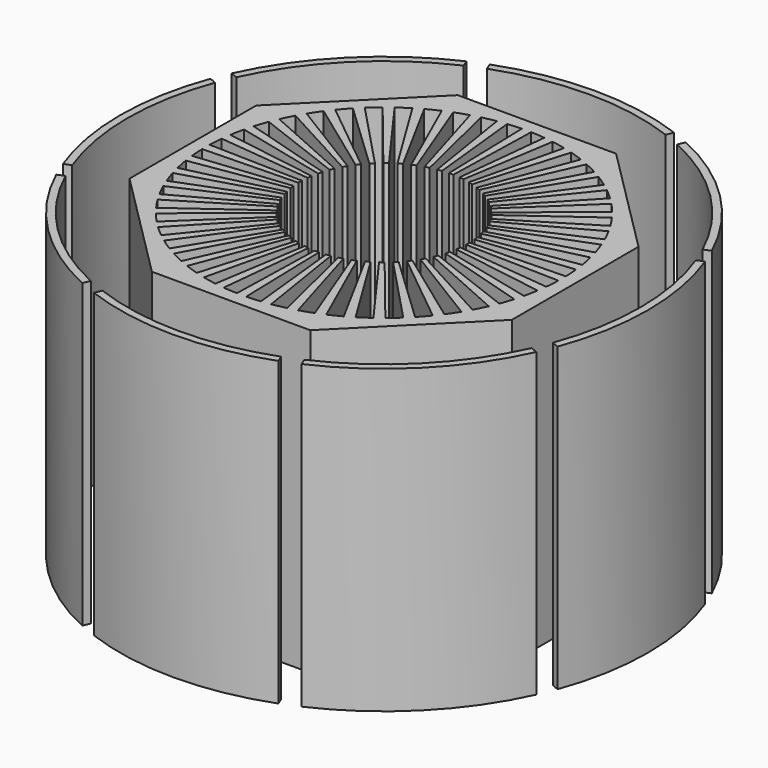
from build123d import *

# Parameters (mm, degrees)
F1_R          = 60
F2_DEPTH      = 50.8
F4_DEPTH      = 50.8
F4_DEPTH_BACK = 50.8
F7_DEPTH      = 50.8
F7_DEPTH_BACK = 50.8
F8_COUNT      = 8


with BuildPart() as f2:
    # F1 (on Top) → F2 (new body, symmetric)
    with BuildSketch(Plane.XY):
        Polygon((26.67, 64.3870757085), (-26.67, 64.3870757085), (-64.3870757085, 26.67), (-64.3870757085, -26.67), (-26.67, -64.3870757085), (26.67, -64.3870757085), (64.3870757085, -26.67), (64.3870757085, 26.67), align=None)
        Circle(F1_R, mode=Mode.SUBTRACT)
    extrude(amount=F2_DEPTH, both=True)

    # F3 (on Top) → F4 (join, two sides)
    with BuildSketch(Plane.XY) as f4_sk:
        with BuildLine():
            ThreePointArc((-0.7394987897, 28.2403194306), (0, 28.25), (0.7394987897, 28.2403194306))
            Line((0.7394987897, 28.2403194306), (1.5706168985, 59.9794394985))
            ThreePointArc((1.5706168985, 59.9794394985), (0, 60), (-1.5706168985, 59.9794394985))
            Line((-1.5706168985, 59.9794394985), (-0.7394987897, 28.2403194306))
        make_face()
        with BuildLine():
            Line((-9.3860679024, 59.2613004357), (-4.4192736374, 27.9021956218))
            ThreePointArc((-4.4192736374, 27.9021956218), (-3.6873649302, 28.0083173338), (-2.9529290873, 28.0952435442))
            Line((-2.9529290873, 28.0952435442), (-6.2717077961, 59.6713137221))
            ThreePointArc((-6.2717077961, 59.6713137221), (-7.8315715332, 59.4866916824), (-9.3860679024, 59.2613004357))
        make_face()
        with BuildLine():
            Line((-17.0409206822, 57.5291840921), (-8.0234334879, 27.08665751))
            ThreePointArc((-8.0234334879, 27.08665751), (-7.3116380241, 27.2874045927), (-6.5948315289, 27.4694502512))
            Line((-6.5948315289, 27.4694502512), (-14.0067218314, 58.3421952239))
            ThreePointArc((-14.0067218314, 58.3421952239), (-15.5291427062, 57.9555495773), (-17.0409206822, 57.5291840921))
        make_face()
        with BuildLine():
            Line((-24.4041985845, 54.8127274586), (-11.4903101669, 25.8076591784))
            ThreePointArc((-11.4903101669, 25.8076591784), (-10.8108069643, 26.0995967934), (-10.1238945747, 26.3736470485))
            Line((-10.1238945747, 26.3736470485), (-21.5020769727, 56.0148255898))
            ThreePointArc((-21.5020769727, 56.0148255898), (-22.9610059419, 55.4327719507), (-24.4041985845, 54.8127274586))
        make_face()
        with BuildLine():
            Line((-31.349913883, 51.1584098612), (-14.7605844532, 24.087084643))
            ThreePointArc((-14.7605844532, 24.087084643), (-14.125, 24.4652176569), (-13.4797349773, 24.8265834327))
            Line((-13.4797349773, 24.8265834327), (-28.6295256156, 52.7290267597))
            ThreePointArc((-28.6295256156, 52.7290267597), (-30, 51.9615242271), (-31.349913883, 51.1584098612))
        make_face()
        with BuildLine():
            Line((-37.759223463, 46.6287576874), (-17.7783010472, 21.9543734112))
            ThreePointArc((-17.7783010472, 21.9543734112), (-17.1975103695, 22.4122318632), (-16.6049333773, 22.8547300911))
            Line((-16.6049333773, 22.8547300911), (-35.2671151375, 48.5410196625))
            ThreePointArc((-35.2671151375, 48.5410196625), (-36.5256857405, 47.6012004175), (-37.759223463, 46.6287576874))
        make_face()
        with BuildLine():
            Line((-43.5224622607, 41.3012745416), (-20.4918259811, 19.4460167633))
            ThreePointArc((-20.4918259811, 19.4460167633), (-19.9757665685, 19.9757665685), (-19.4460167633, 20.4918259811))
            Line((-19.4460167633, 20.4918259811), (-41.3012745416, 43.5224622607))
            ThreePointArc((-41.3012745416, 43.5224622607), (-42.4264068712, 42.4264068712), (-43.5224622607, 41.3012745416))
        make_face()
        with BuildLine():
            Line((-48.5410196625, 35.2671151375), (-22.8547300911, 16.6049333773))
            ThreePointArc((-22.8547300911, 16.6049333773), (-22.4122318632, 17.1975103695), (-21.9543734112, 17.7783010472))
            Line((-21.9543734112, 17.7783010472), (-46.6287576874, 37.759223463))
            ThreePointArc((-46.6287576874, 37.759223463), (-47.6012004175, 36.5256857405), (-48.5410196625, 35.2671151375))
        make_face()
        with BuildLine():
            Line((-52.7290267597, 28.6295256156), (-24.8265834327, 13.4797349773))
            ThreePointArc((-24.8265834327, 13.4797349773), (-24.4652176569, 14.125), (-24.087084643, 14.7605844532))
            Line((-24.087084643, 14.7605844532), (-51.1584098612, 31.349913883))
            ThreePointArc((-51.1584098612, 31.349913883), (-51.9615242271, 30), (-52.7290267597, 28.6295256156))
        make_face()
        with BuildLine():
            Line((-56.0148255898, 21.5020769727), (-26.3736470485, 10.1238945747))
            ThreePointArc((-26.3736470485, 10.1238945747), (-26.0995967934, 10.8108069643), (-25.8076591784, 11.4903101669))
            Line((-25.8076591784, 11.4903101669), (-54.8127274586, 24.4041985845))
            ThreePointArc((-54.8127274586, 24.4041985845), (-55.4327719507, 22.9610059419), (-56.0148255898, 21.5020769727))
        make_face()
        with BuildLine():
            Line((-58.3421952239, 14.0067218314), (-27.4694502512, 6.5948315289))
            ThreePointArc((-27.4694502512, 6.5948315289), (-27.2874045927, 7.3116380241), (-27.08665751, 8.0234334879))
            Line((-27.08665751, 8.0234334879), (-57.5291840921, 17.0409206822))
            ThreePointArc((-57.5291840921, 17.0409206822), (-57.9555495773, 15.5291427062), (-58.3421952239, 14.0067218314))
        make_face()
        with BuildLine():
            Line((-59.6713137221, 6.2717077961), (-28.0952435442, 2.9529290873))
            ThreePointArc((-28.0952435442, 2.9529290873), (-28.0083173338, 3.6873649302), (-27.9021956218, 4.4192736374))
            Line((-27.9021956218, 4.4192736374), (-59.2613004357, 9.3860679024))
            ThreePointArc((-59.2613004357, 9.3860679024), (-59.4866916824, 7.8315715332), (-59.6713137221, 6.2717077961))
        make_face()
        with BuildLine():
            Line((-59.9794394985, -1.5706168985), (-28.2403194306, -0.7394987897))
            ThreePointArc((-28.2403194306, -0.7394987897), (-28.25, 0), (-28.2403194306, 0.7394987897))
            Line((-28.2403194306, 0.7394987897), (-59.9794394985, 1.5706168985))
            ThreePointArc((-59.9794394985, 1.5706168985), (-60, 0), (-59.9794394985, -1.5706168985))
        make_face()
        with BuildLine():
            Line((-59.2613004357, -9.3860679024), (-27.9021956218, -4.4192736374))
            ThreePointArc((-27.9021956218, -4.4192736374), (-28.0083173338, -3.6873649302), (-28.0952435442, -2.9529290873))
            Line((-28.0952435442, -2.9529290873), (-59.6713137221, -6.2717077961))
            ThreePointArc((-59.6713137221, -6.2717077961), (-59.4866916824, -7.8315715332), (-59.2613004357, -9.3860679024))
        make_face()
        with BuildLine():
            Line((-57.5291840921, -17.0409206822), (-27.08665751, -8.0234334879))
            ThreePointArc((-27.08665751, -8.0234334879), (-27.2874045927, -7.3116380241), (-27.4694502512, -6.5948315289))
            Line((-27.4694502512, -6.5948315289), (-58.3421952239, -14.0067218314))
            ThreePointArc((-58.3421952239, -14.0067218314), (-57.9555495773, -15.5291427062), (-57.5291840921, -17.0409206822))
        make_face()
        with BuildLine():
            Line((-54.8127274586, -24.4041985845), (-25.8076591784, -11.4903101669))
            ThreePointArc((-25.8076591784, -11.4903101669), (-26.0995967934, -10.8108069643), (-26.3736470485, -10.1238945747))
            Line((-26.3736470485, -10.1238945747), (-56.0148255898, -21.5020769727))
            ThreePointArc((-56.0148255898, -21.5020769727), (-55.4327719507, -22.9610059419), (-54.8127274586, -24.4041985845))
        make_face()
        with BuildLine():
            Line((-51.1584098612, -31.349913883), (-24.087084643, -14.7605844532))
            ThreePointArc((-24.087084643, -14.7605844532), (-24.4652176569, -14.125), (-24.8265834327, -13.4797349773))
            Line((-24.8265834327, -13.4797349773), (-52.7290267597, -28.6295256156))
            ThreePointArc((-52.7290267597, -28.6295256156), (-51.9615242271, -30), (-51.1584098612, -31.349913883))
        make_face()
        with BuildLine():
            Line((-46.6287576874, -37.759223463), (-21.9543734112, -17.7783010472))
            ThreePointArc((-21.9543734112, -17.7783010472), (-22.4122318632, -17.1975103695), (-22.8547300911, -16.6049333773))
            Line((-22.8547300911, -16.6049333773), (-48.5410196625, -35.2671151375))
            ThreePointArc((-48.5410196625, -35.2671151375), (-47.6012004175, -36.5256857405), (-46.6287576874, -37.759223463))
        make_face()
        with BuildLine():
            Line((-41.3012745416, -43.5224622607), (-19.4460167633, -20.4918259811))
            ThreePointArc((-19.4460167633, -20.4918259811), (-19.9757665685, -19.9757665685), (-20.4918259811, -19.4460167633))
            Line((-20.4918259811, -19.4460167633), (-43.5224622607, -41.3012745416))
            ThreePointArc((-43.5224622607, -41.3012745416), (-42.4264068712, -42.4264068712), (-41.3012745416, -43.5224622607))
        make_face()
        with BuildLine():
            Line((-35.2671151375, -48.5410196625), (-16.6049333773, -22.8547300911))
            ThreePointArc((-16.6049333773, -22.8547300911), (-17.1975103695, -22.4122318632), (-17.7783010472, -21.9543734112))
            Line((-17.7783010472, -21.9543734112), (-37.759223463, -46.6287576874))
            ThreePointArc((-37.759223463, -46.6287576874), (-36.5256857405, -47.6012004175), (-35.2671151375, -48.5410196625))
        make_face()
        with BuildLine():
            Line((-28.6295256156, -52.7290267597), (-13.4797349773, -24.8265834327))
            ThreePointArc((-13.4797349773, -24.8265834327), (-14.125, -24.4652176569), (-14.7605844532, -24.087084643))
            Line((-14.7605844532, -24.087084643), (-31.349913883, -51.1584098612))
            ThreePointArc((-31.349913883, -51.1584098612), (-30, -51.9615242271), (-28.6295256156, -52.7290267597))
        make_face()
        with BuildLine():
            Line((-21.5020769727, -56.0148255898), (-10.1238945747, -26.3736470485))
            ThreePointArc((-10.1238945747, -26.3736470485), (-10.8108069643, -26.0995967934), (-11.4903101669, -25.8076591784))
            Line((-11.4903101669, -25.8076591784), (-24.4041985845, -54.8127274586))
            ThreePointArc((-24.4041985845, -54.8127274586), (-22.9610059419, -55.4327719507), (-21.5020769727, -56.0148255898))
        make_face()
        with BuildLine():
            Line((-14.0067218314, -58.3421952239), (-6.5948315289, -27.4694502512))
            ThreePointArc((-6.5948315289, -27.4694502512), (-7.3116380241, -27.2874045927), (-8.0234334879, -27.08665751))
            Line((-8.0234334879, -27.08665751), (-17.0409206822, -57.5291840921))
            ThreePointArc((-17.0409206822, -57.5291840921), (-15.5291427062, -57.9555495773), (-14.0067218314, -58.3421952239))
        make_face()
        with BuildLine():
            Line((-6.2717077961, -59.6713137221), (-2.9529290873, -28.0952435442))
            ThreePointArc((-2.9529290873, -28.0952435442), (-3.6873649302, -28.0083173338), (-4.4192736374, -27.9021956218))
            Line((-4.4192736374, -27.9021956218), (-9.3860679024, -59.2613004357))
            ThreePointArc((-9.3860679024, -59.2613004357), (-7.8315715332, -59.4866916824), (-6.2717077961, -59.6713137221))
        make_face()
        with BuildLine():
            Line((1.5706168985, -59.9794394985), (0.7394987897, -28.2403194306))
            ThreePointArc((0.7394987897, -28.2403194306), (0, -28.25), (-0.7394987897, -28.2403194306))
            Line((-0.7394987897, -28.2403194306), (-1.5706168985, -59.9794394985))
            ThreePointArc((-1.5706168985, -59.9794394985), (0, -60), (1.5706168985, -59.9794394985))
        make_face()
        with BuildLine():
            Line((9.3860679024, -59.2613004357), (4.4192736374, -27.9021956218))
            ThreePointArc((4.4192736374, -27.9021956218), (3.6873649302, -28.0083173338), (2.9529290873, -28.0952435442))
            Line((2.9529290873, -28.0952435442), (6.2717077961, -59.6713137221))
            ThreePointArc((6.2717077961, -59.6713137221), (7.8315715332, -59.4866916824), (9.3860679024, -59.2613004357))
        make_face()
        with BuildLine():
            Line((17.0409206822, -57.5291840921), (8.0234334879, -27.08665751))
            ThreePointArc((8.0234334879, -27.08665751), (7.3116380241, -27.2874045927), (6.5948315289, -27.4694502512))
            Line((6.5948315289, -27.4694502512), (14.0067218314, -58.3421952239))
            ThreePointArc((14.0067218314, -58.3421952239), (15.5291427062, -57.9555495773), (17.0409206822, -57.5291840921))
        make_face()
        with BuildLine():
            Line((24.4041985845, -54.8127274586), (11.4903101669, -25.8076591784))
            ThreePointArc((11.4903101669, -25.8076591784), (10.8108069643, -26.0995967934), (10.1238945747, -26.3736470485))
            Line((10.1238945747, -26.3736470485), (21.5020769727, -56.0148255898))
            ThreePointArc((21.5020769727, -56.0148255898), (22.9610059419, -55.4327719507), (24.4041985845, -54.8127274586))
        make_face()
        with BuildLine():
            Line((31.349913883, -51.1584098612), (14.7605844532, -24.087084643))
            ThreePointArc((14.7605844532, -24.087084643), (14.125, -24.4652176569), (13.4797349773, -24.8265834327))
            Line((13.4797349773, -24.8265834327), (28.6295256156, -52.7290267597))
            ThreePointArc((28.6295256156, -52.7290267597), (30, -51.9615242271), (31.349913883, -51.1584098612))
        make_face()
        with BuildLine():
            Line((37.759223463, -46.6287576874), (17.7783010472, -21.9543734112))
            ThreePointArc((17.7783010472, -21.9543734112), (17.1975103695, -22.4122318632), (16.6049333773, -22.8547300911))
            Line((16.6049333773, -22.8547300911), (35.2671151375, -48.5410196625))
            ThreePointArc((35.2671151375, -48.5410196625), (36.5256857405, -47.6012004175), (37.759223463, -46.6287576874))
        make_face()
        with BuildLine():
            Line((43.5224622607, -41.3012745416), (20.4918259811, -19.4460167633))
            ThreePointArc((20.4918259811, -19.4460167633), (19.9757665685, -19.9757665685), (19.4460167633, -20.4918259811))
            Line((19.4460167633, -20.4918259811), (41.3012745416, -43.5224622607))
            ThreePointArc((41.3012745416, -43.5224622607), (42.4264068712, -42.4264068712), (43.5224622607, -41.3012745416))
        make_face()
        with BuildLine():
            Line((48.5410196625, -35.2671151375), (22.8547300911, -16.6049333773))
            ThreePointArc((22.8547300911, -16.6049333773), (22.4122318632, -17.1975103695), (21.9543734112, -17.7783010472))
            Line((21.9543734112, -17.7783010472), (46.6287576874, -37.759223463))
            ThreePointArc((46.6287576874, -37.759223463), (47.6012004175, -36.5256857405), (48.5410196625, -35.2671151375))
        make_face()
        with BuildLine():
            Line((52.7290267597, -28.6295256156), (24.8265834327, -13.4797349773))
            ThreePointArc((24.8265834327, -13.4797349773), (24.4652176569, -14.125), (24.087084643, -14.7605844532))
            Line((24.087084643, -14.7605844532), (51.1584098612, -31.349913883))
            ThreePointArc((51.1584098612, -31.349913883), (51.9615242271, -30), (52.7290267597, -28.6295256156))
        make_face()
        with BuildLine():
            Line((56.0148255898, -21.5020769727), (26.3736470485, -10.1238945747))
            ThreePointArc((26.3736470485, -10.1238945747), (26.0995967934, -10.8108069643), (25.8076591784, -11.4903101669))
            Line((25.8076591784, -11.4903101669), (54.8127274586, -24.4041985845))
            ThreePointArc((54.8127274586, -24.4041985845), (55.4327719507, -22.9610059419), (56.0148255898, -21.5020769727))
        make_face()
        with BuildLine():
            Line((58.3421952239, -14.0067218314), (27.4694502512, -6.5948315289))
            ThreePointArc((27.4694502512, -6.5948315289), (27.2874045927, -7.3116380241), (27.08665751, -8.0234334879))
            Line((27.08665751, -8.0234334879), (57.5291840921, -17.0409206822))
            ThreePointArc((57.5291840921, -17.0409206822), (57.9555495773, -15.5291427062), (58.3421952239, -14.0067218314))
        make_face()
        with BuildLine():
            Line((59.6713137221, -6.2717077961), (28.0952435442, -2.9529290873))
            ThreePointArc((28.0952435442, -2.9529290873), (28.0083173338, -3.6873649302), (27.9021956218, -4.4192736374))
            Line((27.9021956218, -4.4192736374), (59.2613004357, -9.3860679024))
            ThreePointArc((59.2613004357, -9.3860679024), (59.4866916824, -7.8315715332), (59.6713137221, -6.2717077961))
        make_face()
        with BuildLine():
            Line((59.9794394985, 1.5706168985), (28.2403194306, 0.7394987897))
            ThreePointArc((28.2403194306, 0.7394987897), (28.25, 0), (28.2403194306, -0.7394987897))
            Line((28.2403194306, -0.7394987897), (59.9794394985, -1.5706168985))
            ThreePointArc((59.9794394985, -1.5706168985), (60, 0), (59.9794394985, 1.5706168985))
        make_face()
        with BuildLine():
            Line((59.2613004357, 9.3860679024), (27.9021956218, 4.4192736374))
            ThreePointArc((27.9021956218, 4.4192736374), (28.0083173338, 3.6873649302), (28.0952435442, 2.9529290873))
            Line((28.0952435442, 2.9529290873), (59.6713137221, 6.2717077961))
            ThreePointArc((59.6713137221, 6.2717077961), (59.4866916824, 7.8315715332), (59.2613004357, 9.3860679024))
        make_face()
        with BuildLine():
            Line((57.5291840921, 17.0409206822), (27.08665751, 8.0234334879))
            ThreePointArc((27.08665751, 8.0234334879), (27.2874045927, 7.3116380241), (27.4694502512, 6.5948315289))
            Line((27.4694502512, 6.5948315289), (58.3421952239, 14.0067218314))
            ThreePointArc((58.3421952239, 14.0067218314), (57.9555495773, 15.5291427062), (57.5291840921, 17.0409206822))
        make_face()
        with BuildLine():
            Line((54.8127274586, 24.4041985845), (25.8076591784, 11.4903101669))
            ThreePointArc((25.8076591784, 11.4903101669), (26.0995967934, 10.8108069643), (26.3736470485, 10.1238945747))
            Line((26.3736470485, 10.1238945747), (56.0148255898, 21.5020769727))
            ThreePointArc((56.0148255898, 21.5020769727), (55.4327719507, 22.9610059419), (54.8127274586, 24.4041985845))
        make_face()
        with BuildLine():
            Line((51.1584098612, 31.349913883), (24.087084643, 14.7605844532))
            ThreePointArc((24.087084643, 14.7605844532), (24.4652176569, 14.125), (24.8265834327, 13.4797349773))
            Line((24.8265834327, 13.4797349773), (52.7290267597, 28.6295256156))
            ThreePointArc((52.7290267597, 28.6295256156), (51.9615242271, 30), (51.1584098612, 31.349913883))
        make_face()
        with BuildLine():
            Line((46.6287576874, 37.759223463), (21.9543734112, 17.7783010472))
            ThreePointArc((21.9543734112, 17.7783010472), (22.4122318632, 17.1975103695), (22.8547300911, 16.6049333773))
            Line((22.8547300911, 16.6049333773), (48.5410196625, 35.2671151375))
            ThreePointArc((48.5410196625, 35.2671151375), (47.6012004175, 36.5256857405), (46.6287576874, 37.759223463))
        make_face()
        with BuildLine():
            Line((41.3012745416, 43.5224622607), (19.4460167633, 20.4918259811))
            ThreePointArc((19.4460167633, 20.4918259811), (19.9757665685, 19.9757665685), (20.4918259811, 19.4460167633))
            Line((20.4918259811, 19.4460167633), (43.5224622607, 41.3012745416))
            ThreePointArc((43.5224622607, 41.3012745416), (42.4264068712, 42.4264068712), (41.3012745416, 43.5224622607))
        make_face()
        with BuildLine():
            Line((35.2671151375, 48.5410196625), (16.6049333773, 22.8547300911))
            ThreePointArc((16.6049333773, 22.8547300911), (17.1975103695, 22.4122318632), (17.7783010472, 21.9543734112))
            Line((17.7783010472, 21.9543734112), (37.759223463, 46.6287576874))
            ThreePointArc((37.759223463, 46.6287576874), (36.5256857405, 47.6012004175), (35.2671151375, 48.5410196625))
        make_face()
        with BuildLine():
            Line((28.6295256156, 52.7290267597), (13.4797349773, 24.8265834327))
            ThreePointArc((13.4797349773, 24.8265834327), (14.125, 24.4652176569), (14.7605844532, 24.087084643))
            Line((14.7605844532, 24.087084643), (31.349913883, 51.1584098612))
            ThreePointArc((31.349913883, 51.1584098612), (30, 51.9615242271), (28.6295256156, 52.7290267597))
        make_face()
        with BuildLine():
            Line((21.5020769727, 56.0148255898), (10.1238945747, 26.3736470485))
            ThreePointArc((10.1238945747, 26.3736470485), (10.8108069643, 26.0995967934), (11.4903101669, 25.8076591784))
            Line((11.4903101669, 25.8076591784), (24.4041985845, 54.8127274586))
            ThreePointArc((24.4041985845, 54.8127274586), (22.9610059419, 55.4327719507), (21.5020769727, 56.0148255898))
        make_face()
        with BuildLine():
            Line((14.0067218314, 58.3421952239), (6.5948315289, 27.4694502512))
            ThreePointArc((6.5948315289, 27.4694502512), (7.3116380241, 27.2874045927), (8.0234334879, 27.08665751))
            Line((8.0234334879, 27.08665751), (17.0409206822, 57.5291840921))
            ThreePointArc((17.0409206822, 57.5291840921), (15.5291427062, 57.9555495773), (14.0067218314, 58.3421952239))
        make_face()
        with BuildLine():
            Line((6.2717077961, 59.6713137221), (2.9529290873, 28.0952435442))
            ThreePointArc((2.9529290873, 28.0952435442), (3.6873649302, 28.0083173338), (4.4192736374, 27.9021956218))
            Line((4.4192736374, 27.9021956218), (9.3860679024, 59.2613004357))
            ThreePointArc((9.3860679024, 59.2613004357), (7.8315715332, 59.4866916824), (6.2717077961, 59.6713137221))
        make_face()
    extrude(amount=F4_DEPTH)
    extrude(f4_sk.sketch, amount=-F4_DEPTH_BACK)


with BuildPart() as f7:
    # F6 (on Top) → F7 (new body, two sides)
    with BuildSketch(Plane.XY) as f7_sk:
        with BuildLine():
            Line((-30.0928812264, -80.9473168147), (-31.0655359146, -83.2955129544))
            ThreePointArc((-31.0655359146, -83.2955129544), (0, -88.9), (31.0655359146, -83.2955129544))
            Line((31.0655359146, -83.2955129544), (30.0928812264, -80.9473168147))
            ThreePointArc((30.0928812264, -80.9473168147), (0, -86.36), (-30.0928812264, -80.9473168147))
        make_face()
    extrude(amount=-F7_DEPTH)
    extrude(f7_sk.sketch, amount=F7_DEPTH_BACK)


with BuildPart() as f8_1:
    # F8: instance of F7
    add(f7.part.rotate(Axis((0, 0, 0), (0, 0, 1)), 1 * 360 / F8_COUNT))


with BuildPart() as f8_2:
    # F8: instance of F7
    add(f7.part.rotate(Axis((0, 0, 0), (0, 0, 1)), 2 * 360 / F8_COUNT))


with BuildPart() as f8_3:
    # F8: instance of F7
    add(f7.part.rotate(Axis((0, 0, 0), (0, 0, 1)), 3 * 360 / F8_COUNT))


with BuildPart() as f8_4:
    # F8: instance of F7
    add(f7.part.rotate(Axis((0, 0, 0), (0, 0, 1)), 4 * 360 / F8_COUNT))


with BuildPart() as f8_5:
    # F8: instance of F7
    add(f7.part.rotate(Axis((0, 0, 0), (0, 0, 1)), 5 * 360 / F8_COUNT))


with BuildPart() as f8_6:
    # F8: instance of F7
    add(f7.part.rotate(Axis((0, 0, 0), (0, 0, 1)), 6 * 360 / F8_COUNT))


with BuildPart() as f8_7:
    # F8: instance of F7
    add(f7.part.rotate(Axis((0, 0, 0), (0, 0, 1)), 7 * 360 / F8_COUNT))


solid = Compound([f2.part, f7.part, f8_1.part, f8_2.part, f8_3.part, f8_4.part, f8_5.part, f8_6.part, f8_7.part])
